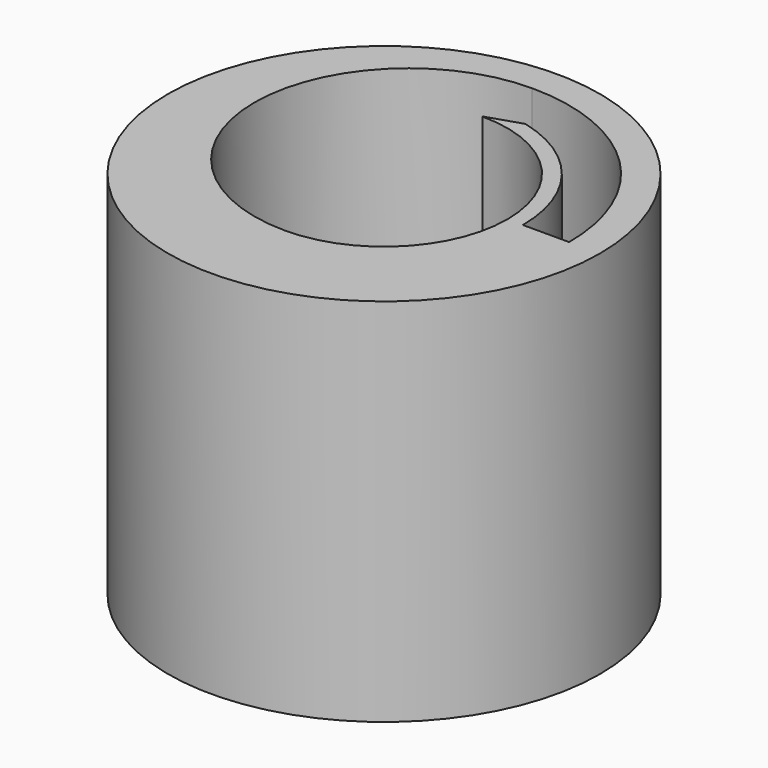
from build123d import *

# Parameters (mm, degrees)
F0_R        = 44.45
F1_DEPTH    = 76.2
F3_DEPTH    = 38.1
F4_T1_DEPTH = 56.0791508125
F5_DEPTH    = 76.201


# Not quite as in the source:
# - a fillet or chamfer that OpenCascade refuses, or shapes differently, is made with other operations: its cross-section is extruded or revolved along the edge and cut away or added


with BuildPart() as f1:
    # F0 (on Top) → F1 (new body)
    with BuildSketch(Plane.XY):
        Circle(F0_R)
    extrude(amount=F1_DEPTH)

    # F2 (on face) → F3 (cut)
    with BuildSketch(Plane.XY.offset(76.2)):
        with BuildLine():
            Line((0, 28.575), (0, 38.1))
            ThreePointArc((0, 38.1), (-28.175329967, 20.986026826), (-25.976370723, -11.90625))
            ThreePointArc((-25.976370723, -11.90625), (-24.0494461345, 15.4322637881), (0, 28.575))
        make_face()
        with BuildLine():
            ThreePointArc((0, 28.575), (-24.0494461345, 15.4322637881), (-25.976370723, -11.90625))
            ThreePointArc((-25.976370723, -11.90625), (-14.636026826, -21.825329967), (0, -25.4))
            ThreePointArc((0, -25.4), (-25.4, 0), (0, 25.4))
            Line((0, 25.4), (0, 28.575))
        make_face()
        with BuildLine():
            ThreePointArc((0, 25.4), (-25.4, 0), (0, -25.4))
            Line((0, -25.4), (0, -2.38125))
            ThreePointArc((0, -2.38125), (-2.38125, 0), (0, 2.38125))
            Line((0, 2.38125), (0, 25.4))
        make_face()
        with BuildLine():
            Line((0, -2.38125), (0, -25.4))
            ThreePointArc((0, -25.4), (17.9605122421, -17.9605122421), (25.4, 0))
            ThreePointArc((25.4, 0), (17.9605122421, 17.9605122421), (0, 25.4))
            Line((0, 25.4), (0, 2.38125))
            ThreePointArc((0, 2.38125), (1.6837980227, 1.6837980227), (2.38125, 0))
            ThreePointArc((2.38125, 0), (1.6837980227, -1.6837980227), (0, -2.38125))
        make_face()
        with BuildLine():
            Line((28.575, 0), (38.1, 0))
            ThreePointArc((38.1, 0), (26.9407683632, 26.9407683632), (0, 38.1))
            Line((0, 38.1), (0, 28.575))
            ThreePointArc((0, 28.575), (20.2055762724, 20.2055762724), (28.575, 0))
        make_face()
    extrude(amount=-F3_DEPTH, mode=Mode.SUBTRACT)

    # F4: chamfer of 6.35 x 2.3112109876 on 1 edges, made by hand

    # F4_s2 → F4_t1 (cut)
    with BuildSketch(Plane.XY.offset(38.1)):
        with BuildLine():
            Line((0, 25.4845857979), (6.9087994087, 27.7272269751))
            ThreePointArc((6.9087994087, 27.7272269751), (3.5951834098, 28.3479325745), (0, 28.575))
            Line((0, 28.575), (0, 25.4845857979))
        make_face()
    extrude(amount=F4_T1_DEPTH, mode=Mode.SUBTRACT)

    # F5 (cut, through all): a face of the model
    f5_faces = [f1.faces().sort_by_distance(p)[0] for p in [
        (0, 0, 76.2),
    ]]
    extrude(f5_faces, amount=-F5_DEPTH, mode=Mode.SUBTRACT)


solid = f1.part
